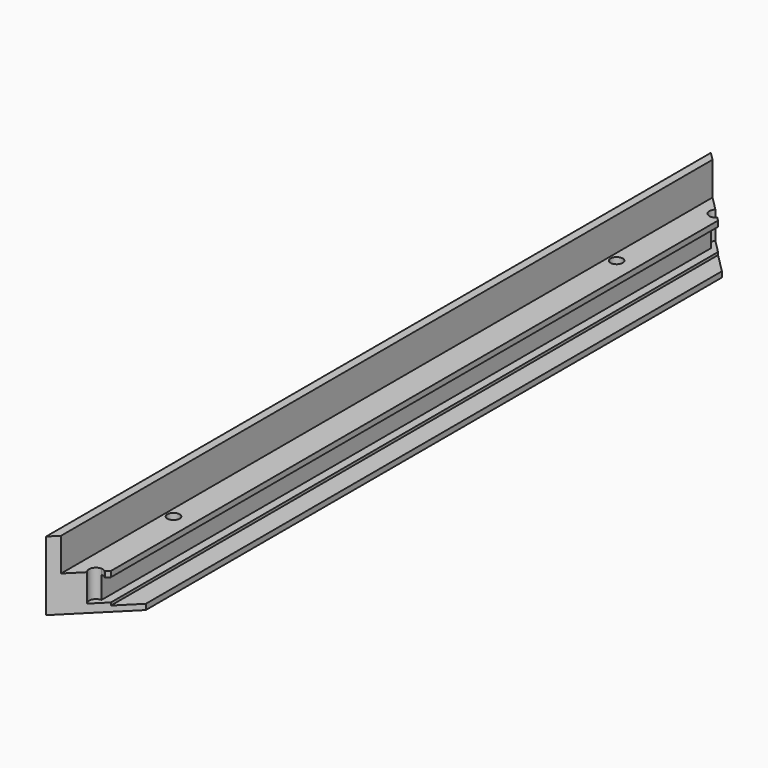
from build123d import *

# Parameters (mm, degrees)
F0_W     = 3
F0_H     = 12
F0_W_2   = 7
F0_H_2   = 1
F1_DEPTH = 150
F3_D     = 4.4
F3_DEPTH = 10.4
F3_TIP   = 1.3218933619
F4_SIZE  = 19.99999
F6_DEPTH = 8


# Not quite as in the source:
# - a fillet or chamfer is up to 0.001 mm smaller than in the source, because OpenCascade refuses the exact size


with BuildPart() as f1:
    # F0 (on Front) → F1 (new body)
    with BuildSketch(Plane.XZ):
        with Locations((-8.5, 8)):
            Rectangle(F0_W, F0_H)
        Polygon((-10, 0), (0, 0), (3, 0), (3, 2), (-7, 2), (-10, 2), align=None)
        Polygon((0, -8), (0, 0), (-10, 0), (-10, -10), (0, -10), align=None)
        Polygon((0, -10), (-10, -10), (-10, -11), (10, -11), (10, -10), (3, -10), align=None)
        with Locations((6.5, -9.5)):
            Rectangle(F0_W_2, F0_H_2)
        Polygon((3, -8), (0, -8), (0, -10), (3, -10), (3, -9), align=None)
    extrude(amount=F1_DEPTH)

    # F3
    with Locations(Plane.XY.offset(2)):
        with Locations((-4, -100)):
            Hole(F3_D / 2, depth=F3_DEPTH)
            with Locations((0, 0, -(F3_DEPTH + F3_TIP / 2))):  # 118° drill point
                Cone(0, F3_D / 2, F3_TIP, mode=Mode.SUBTRACT)

    # F4 (size 20 in the source; OpenCascade refuses exactly that, so slightly less here)
    f4_edges = [f1.edges().sort_by_distance(p)[0] for p in [
        (10, -150, -10),
    ]]
    chamfer(f4_edges, length=F4_SIZE)

    # F5 (on face) → F6 (cut, symmetric)
    with BuildSketch(Plane(origin=(0, 0, 0), x_dir=(1, 0, 0), z_dir=(0, 0, -1))):
        with BuildLine():
            ThreePointArc((1.767771953, 138.232238047), (2.3097001843, 139.0432946855), (2.5, 140))
            ThreePointArc((2.5, 140), (-1.767766953, 141.767766953), (0, 137.5))
            Line((0, 137.5), (0, 140.00001))
            Line((0, 140.00001), (1.767771953, 138.232238047))
        make_face()
        with BuildLine():
            Line((0, 140.00001), (0, 137.5))
            ThreePointArc((0, 137.5), (0.9567118473, 137.6903025217), (1.767771953, 138.232238047))
            Line((1.767771953, 138.232238047), (0, 140.00001))
        make_face()
    extrude(amount=F6_DEPTH, both=True, mode=Mode.SUBTRACT)

    # F7: F1 across face


with BuildPart() as f1_1:
    add(f1.part)
    add(f1.part.mirror(Plane(origin=(-4.3205128205, 0, -2.6487179487), x_dir=(1, 0, 0), z_dir=(0, 1, 0))))


solid = f1_1.part
